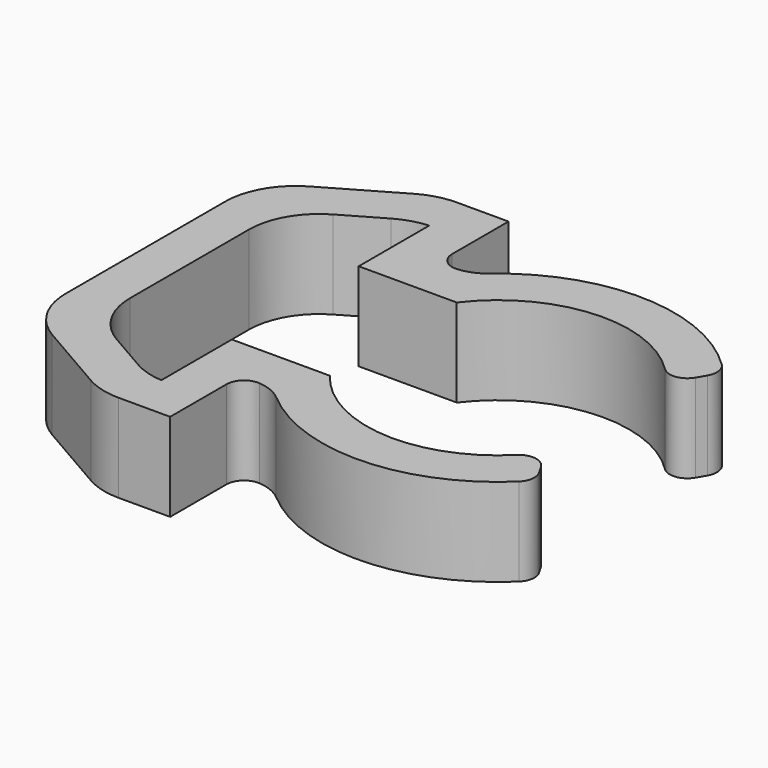
from build123d import *

# Parameters (mm, degrees)
F1_DEPTH     = 6.35
F2_T1_DEPTH  = 6.35
F2_T3_DEPTH  = 6.35
F2_T5_DEPTH  = 6.35
F2_T7_DEPTH  = 6.35
F2_T9_DEPTH  = 13.1559094878
F2_T11_DEPTH = 21.0146968374
F2_T13_DEPTH = 21.0146968374
F2_T15_DEPTH = 13.1559094878
F3_R         = 3.175
F4_R         = 1.27
F5_R         = 1.27


# Not quite as in the source:
# - a fillet or chamfer that OpenCascade refuses, or shapes differently, is made with other operations: its cross-section is extruded or revolved along the edge and cut away or added


with BuildPart() as f1:
    # F0 (on Top) → F1 (new body)
    with BuildSketch(Plane.XY):
        with BuildLine():
            ThreePointArc((7.7709057387, -5.3975), (0.1961534845, -9.4594664786), (-7.5404746038, -5.715))
            Line((-7.5404746038, -5.715), (-14.605, -5.715))
            Line((-14.605, -5.715), (-14.605, -12.065))
            Line((-14.605, -12.065), (-15.659261314, -12.065))
            Line((-15.659261314, -12.065), (-22.225, -8.2742690022))
            Line((-22.225, -8.2742690022), (-22.225, 8.2742690022))
            Line((-22.225, 8.2742690022), (-15.659261314, 12.065))
            Line((-15.659261314, 12.065), (-14.605, 12.065))
            Line((-14.605, 12.065), (-14.605, 5.715))
            Line((-14.605, 5.715), (-7.5404746038, 5.715))
            ThreePointArc((-7.5404746038, 5.715), (0.1961534845, 9.4594664786), (7.7709057387, 5.3975))
            Line((7.7709057387, 5.3975), (9.5126338349, 8.4142615555))
            ThreePointArc((9.5126338349, 8.4142615555), (0.3250359785, 12.6958399333), (-9.0696141042, 8.89))
            Line((-9.0696141042, 8.89), (-11.43, 8.89))
            Line((-11.43, 8.89), (-11.43, 15.24))
            Line((-11.43, 15.24), (-16.51, 15.24))
            Line((-16.51, 15.24), (-25.4, 10.1073561069))
            Line((-25.4, 10.1073561069), (-25.4, -10.1073561069))
            Line((-25.4, -10.1073561069), (-16.51, -15.24))
            Line((-16.51, -15.24), (-11.43, -15.24))
            Line((-11.43, -15.24), (-11.43, -8.89))
            Line((-11.43, -8.89), (-9.0696141042, -8.89))
            ThreePointArc((-9.0696141042, -8.89), (0.3250359785, -12.6958399333), (9.5126338349, -8.4142615555))
            Line((9.5126338349, -8.4142615555), (7.7709057387, -5.3975))
        make_face()
    extrude(amount=F1_DEPTH)

    # F2: fillet of radius 5.08 on 8 edges, made by hand

    # F2_s2 → F2_t1 (join)
    with BuildSketch(Plane.XY):
        with BuildLine():
            ThreePointArc((-14.605, -12.065), (-15.7512023765, -11.857721614), (-16.8200610521, -11.3948119587))
            Line((-16.8200610521, -11.3948119587), (-15.659261314, -12.065))
            Line((-15.659261314, -12.065), (-14.605, -12.065))
        make_face()
    extrude(amount=F2_T1_DEPTH)

    # F2_s4 → F2_t3 (join)
    with BuildSketch(Plane.XY):
        with BuildLine():
            ThreePointArc((-19.685, -9.740738686), (-21.5444090512, -7.8813296347), (-22.225, -5.3413296347))
            Line((-22.225, -5.3413296347), (-22.225, -8.2742690022))
            Line((-22.225, -8.2742690022), (-19.685, -9.740738686))
        make_face()
    extrude(amount=F2_T3_DEPTH)

    # F2_s6 → F2_t5 (join)
    with BuildSketch(Plane.XY):
        with BuildLine():
            ThreePointArc((-22.225, 5.3413296347), (-21.5444090512, 7.8813296347), (-19.685, 9.740738686))
            Line((-19.685, 9.740738686), (-22.225, 8.2742690022))
            Line((-22.225, 8.2742690022), (-22.225, 5.3413296347))
        make_face()
    extrude(amount=F2_T5_DEPTH)

    # F2_s8 → F2_t7 (join)
    with BuildSketch(Plane.XY):
        with BuildLine():
            ThreePointArc((-16.8200610521, 11.3948119587), (-15.7512023765, 11.857721614), (-14.605, 12.065))
            Line((-14.605, 12.065), (-15.659261314, 12.065))
            Line((-15.659261314, 12.065), (-16.8200610521, 11.3948119587))
        make_face()
    extrude(amount=F2_T7_DEPTH)

    # F2_s10 → F2_t9 (cut)
    with BuildSketch(Plane.XY.offset(-3.4029547439)):
        with BuildLine():
            ThreePointArc((-15.1488181024, 15.24), (-16.4636188516, 15.0669031975), (-17.6888181024, 14.5594090512))
            Line((-17.6888181024, 14.5594090512), (-16.51, 15.24))
            Line((-16.51, 15.24), (-15.1488181024, 15.24))
        make_face()
    extrude(amount=F2_T9_DEPTH, mode=Mode.SUBTRACT)

    # F2_s12 → F2_t11 (cut)
    with BuildSketch(Plane.XY.offset(-7.3323484187)):
        with BuildLine():
            ThreePointArc((-25.4, 7.1744167394), (-24.7194090512, 9.7144167394), (-22.86, 11.5738257906))
            Line((-22.86, 11.5738257906), (-25.4, 10.1073561069))
            Line((-25.4, 10.1073561069), (-25.4, 7.1744167394))
        make_face()
    extrude(amount=F2_T11_DEPTH, mode=Mode.SUBTRACT)

    # F2_s14 → F2_t13 (cut)
    with BuildSketch(Plane.XY.offset(-7.3323484187)):
        with BuildLine():
            ThreePointArc((-22.86, -11.5738257906), (-24.7194090512, -9.7144167394), (-25.4, -7.1744167394))
            Line((-25.4, -7.1744167394), (-25.4, -10.1073561069))
            Line((-25.4, -10.1073561069), (-22.86, -11.5738257906))
        make_face()
    extrude(amount=F2_T13_DEPTH, mode=Mode.SUBTRACT)

    # F2_s16 → F2_t15 (cut)
    with BuildSketch(Plane.XY.offset(-3.4029547439)):
        with BuildLine():
            ThreePointArc((-15.1488181024, -15.24), (-16.4636188516, -15.0669031975), (-17.6888181024, -14.5594090512))
            Line((-17.6888181024, -14.5594090512), (-16.51, -15.24))
            Line((-16.51, -15.24), (-15.1488181024, -15.24))
        make_face()
    extrude(amount=F2_T15_DEPTH, mode=Mode.SUBTRACT)

    # F3
    f3_edges = [f1.edges().sort_by_distance(p)[0] for p in [
        (-9.069614, 8.89, 3.175),
        (-9.069614, -8.89, 3.175),
    ]]
    fillet(f3_edges, radius=F3_R)

    # F4
    f4_edges = [f1.edges().sort_by_distance(p)[0] for p in [
        (-11.43, -8.89, 3.175),
        (-11.43, 8.89, 3.175),
    ]]
    fillet(f4_edges, radius=F4_R)

    # F5
    f5_edges = [f1.edges().sort_by_distance(p)[0] for p in [
        (7.770906, -5.3975, 3.175),
        (9.512634, -8.414262, 3.175),
        (9.512634, 8.414262, 3.175),
        (7.770906, 5.3975, 3.175),
    ]]
    fillet(f5_edges, radius=F5_R)


solid = f1.part
